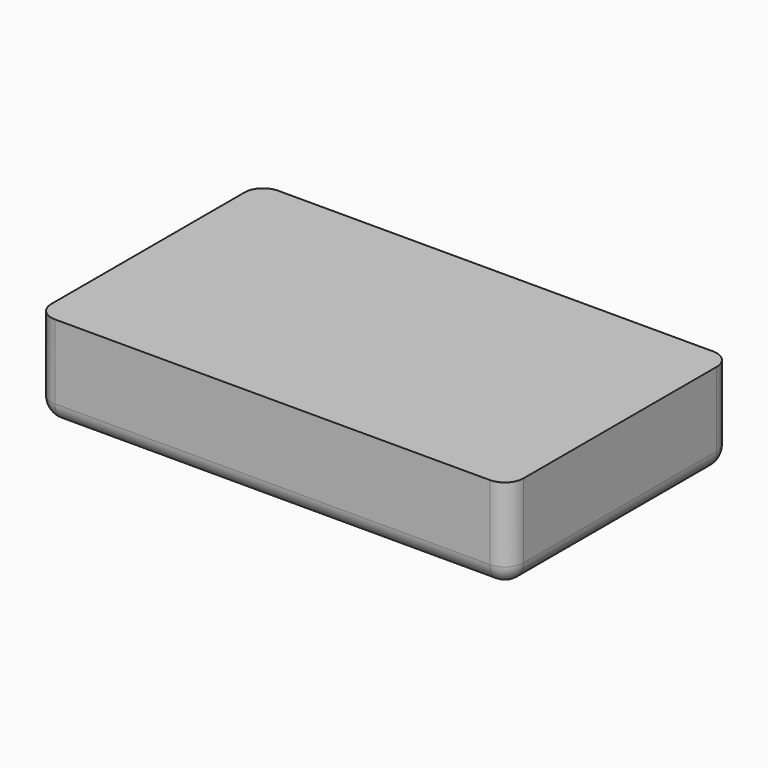
from build123d import *

# Parameters (mm, degrees)
F0_W         = 50.8
F0_H         = 30
F1_DEPTH     = 10
F2_W         = 3
F2_H         = 26
F2_W_2       = 11.5
F2_H_2       = 1.5
F3_DEPTH     = 8
F4_T1_DEPTH  = 13
F4_T3_DEPTH  = 26
F4_T5_DEPTH  = 46.8
F4_S9_W      = 2
F4_S9_H      = 2
F4_T10_DEPTH = 2
F4_S15_W     = 2
F4_S15_H     = 2
F4_T16_DEPTH = 2
F4_S21_W     = 2
F4_S21_H     = 2
F4_T22_DEPTH = 2
F4_S27_W     = 2
F4_S27_H     = 2
F4_T28_DEPTH = 2


# Not quite as in the source:
# - a fillet or chamfer that OpenCascade refuses, or shapes differently, is made with other operations: its cross-section is extruded or revolved along the edge and cut away or added


with BuildPart() as f1:
    # F0 (on Top) → F1 (new body)
    with BuildSketch(Plane.XY):
        Rectangle(F0_W, F0_H)
    extrude(amount=F1_DEPTH)

    # F2 (on Top) → F3 (cut)
    with BuildSketch(Plane.XY):
        with Locations((-7.3340023962, 0.1232437862)):
            Rectangle(F2_W, F2_H)
        with Locations((-11.9503338486, 0.091059359)):
            Rectangle(F2_W, F2_H)
        with Locations((-16.8786235154, 0.0321844273)):
            Rectangle(F2_W, F2_H)
        with Locations((-21.4949549678, 0)):
            Rectangle(F2_W, F2_H)
        with Locations((5.75, 4.3395428155)):
            Rectangle(F2_W_2, F2_H_2)
        with Locations((5.75, 6.9914316775)):
            Rectangle(F2_W_2, F2_H_2)
        with Locations((5.75, 9.7213549241)):
            Rectangle(F2_W_2, F2_H_2)
        with Locations((5.75, 12.3732437862)):
            Rectangle(F2_W_2, F2_H_2)
        with Locations((5.75, 1.6359822841)):
            Rectangle(F2_W_2, F2_H_2)
        with Locations((5.75, -1.0159065779)):
            Rectangle(F2_W_2, F2_H_2)
        with Locations((5.75, -3.7458298245)):
            Rectangle(F2_W_2, F2_H_2)
        with Locations((5.75, -6.3977186866)):
            Rectangle(F2_W_2, F2_H_2)
    extrude(amount=F3_DEPTH, mode=Mode.SUBTRACT)

    # F4: fillet of radius 2 on 8 edges, made by hand

    # F4_s2 → F4_t1 (cut)
    with BuildSketch(Plane.XY.offset(2)):
        with BuildLine():
            ThreePointArc((25.4, 13), (24.8142135624, 14.4142135624), (23.4, 15))
            Line((23.4, 15), (25.4, 15))
            Line((25.4, 15), (25.4, 13))
        make_face()
        with BuildLine():
            ThreePointArc((25.4, -13), (24.8142135624, -14.4142135624), (23.4, -15))
            Line((23.4, -15), (25.4, -15))
            Line((25.4, -15), (25.4, -13))
        make_face()
        with BuildLine():
            ThreePointArc((-23.4, -15), (-24.8142135624, -14.4142135624), (-25.4, -13))
            Line((-25.4, -13), (-25.4, -15))
            Line((-25.4, -15), (-23.4, -15))
        make_face()
        with BuildLine():
            ThreePointArc((-23.4, 15), (-24.8142135624, 14.4142135624), (-25.4, 13))
            Line((-25.4, 13), (-25.4, 15))
            Line((-25.4, 15), (-23.4, 15))
        make_face()
    extrude(amount=F4_T1_DEPTH, mode=Mode.SUBTRACT)

    # F4_s4 → F4_t3 (cut)
    with BuildSketch(Plane.XZ.offset(-13)):
        with BuildLine():
            ThreePointArc((25.4, 2), (24.8142135624, 0.5857864376), (23.4, 0))
            Line((23.4, 0), (25.4, 0))
            Line((25.4, 0), (25.4, 2))
        make_face()
        with BuildLine():
            ThreePointArc((-23.4, 0), (-24.8142135624, 0.5857864376), (-25.4, 2))
            Line((-25.4, 2), (-25.4, 0))
            Line((-25.4, 0), (-23.4, 0))
        make_face()
    extrude(amount=F4_T3_DEPTH, mode=Mode.SUBTRACT)

    # F4_s6 → F4_t5 (cut)
    with BuildSketch(Plane.YZ.offset(-23.4)):
        with BuildLine():
            ThreePointArc((-15, 2), (-14.4142135624, 0.5857864376), (-13, 0))
            Line((-13, 0), (-15, 0))
            Line((-15, 0), (-15, 2))
        make_face()
        with BuildLine():
            ThreePointArc((15, 2), (14.4142135624, 0.5857864376), (13, 0))
            Line((13, 0), (15, 0))
            Line((15, 0), (15, 2))
        make_face()
    extrude(amount=F4_T5_DEPTH, mode=Mode.SUBTRACT)


with BuildPart() as f4_tool8:
    # F4_s9 → F4_t10 (new body)
    with BuildSketch(Plane.YZ.offset(23.4)):
        with Locations((14, 1)):
            Rectangle(F4_S9_W, F4_S9_H)
    extrude(amount=F4_T10_DEPTH)

    # F4_s11 → F4_t12 (revolve, cut)
    with BuildSketch(Plane(origin=(23.4, 13, 2), x_dir=(0, -0.7071067812, 0.7071067812), z_dir=(0, 0.7071067812, 0.7071067812))):
        with BuildLine():
            ThreePointArc((0, -2), (2, 0), (0, 2))
            Line((0, 2), (0, -2))
        make_face()
    revolve(axis=Axis((23.4, 13, 2), (1, 0, 0)), mode=Mode.SUBTRACT)


with BuildPart() as f1_1:
    add(f1.part)

    # F4_t7: cut F4_tool8
    add(f4_tool8.part, mode=Mode.SUBTRACT)


with BuildPart() as f4_tool14:
    # F4_s15 → F4_t16 (new body)
    with BuildSketch(Plane.YZ.offset(23.4)):
        with Locations((-14, 1)):
            Rectangle(F4_S15_W, F4_S15_H)
    extrude(amount=F4_T16_DEPTH)

    # F4_s17 → F4_t18 (revolve, cut)
    with BuildSketch(Plane(origin=(23.4, -13, 2), x_dir=(0, 0.7071067812, 0.7071067812), z_dir=(0, 0.7071067812, -0.7071067812))):
        with BuildLine():
            ThreePointArc((0, -2), (2, 0), (0, 2))
            Line((0, 2), (0, -2))
        make_face()
    revolve(axis=Axis((23.4, -13, 2), (1, 0, 0)), mode=Mode.SUBTRACT)


with BuildPart() as f1_2:
    add(f1_1.part)

    # F4_t13: cut F4_tool14
    add(f4_tool14.part, mode=Mode.SUBTRACT)


with BuildPart() as f4_tool20:
    # F4_s21 → F4_t22 (new body)
    with BuildSketch(Plane.XZ.offset(13)):
        with Locations((-24.4, 1)):
            Rectangle(F4_S21_W, F4_S21_H)
    extrude(amount=F4_T22_DEPTH)

    # F4_s23 → F4_t24 (revolve, cut)
    with BuildSketch(Plane(origin=(-23.4, -13, 2), x_dir=(0.7071067812, 0, 0.7071067812), z_dir=(0.7071067812, 0, -0.7071067812))):
        with BuildLine():
            ThreePointArc((0, -2), (2, 0), (0, 2))
            Line((0, 2), (0, -2))
        make_face()
    revolve(axis=Axis((-23.4, -13, 2), (0, -1, 0)), mode=Mode.SUBTRACT)


with BuildPart() as f1_3:
    add(f1_2.part)

    # F4_t19: cut F4_tool20
    add(f4_tool20.part, mode=Mode.SUBTRACT)


with BuildPart() as f4_tool26:
    # F4_s27 → F4_t28 (new body)
    with BuildSketch(Plane.XZ.offset(-13)):
        with Locations((-24.4, 1)):
            Rectangle(F4_S27_W, F4_S27_H)
    extrude(amount=-F4_T28_DEPTH)

    # F4_s29 → F4_t30 (revolve, cut)
    with BuildSketch(Plane(origin=(-23.4, 13, 2), x_dir=(0.7071067812, 0, 0.7071067812), z_dir=(-0.7071067812, 0, 0.7071067812))):
        with BuildLine():
            ThreePointArc((0, -2), (2, 0), (0, 2))
            Line((0, 2), (0, -2))
        make_face()
    revolve(axis=Axis((-23.4, 13, 2), (0, 1, 0)), mode=Mode.SUBTRACT)


with BuildPart() as f1_4:
    add(f1_3.part)

    # F4_t25: cut F4_tool26
    add(f4_tool26.part, mode=Mode.SUBTRACT)


solid = f1_4.part
